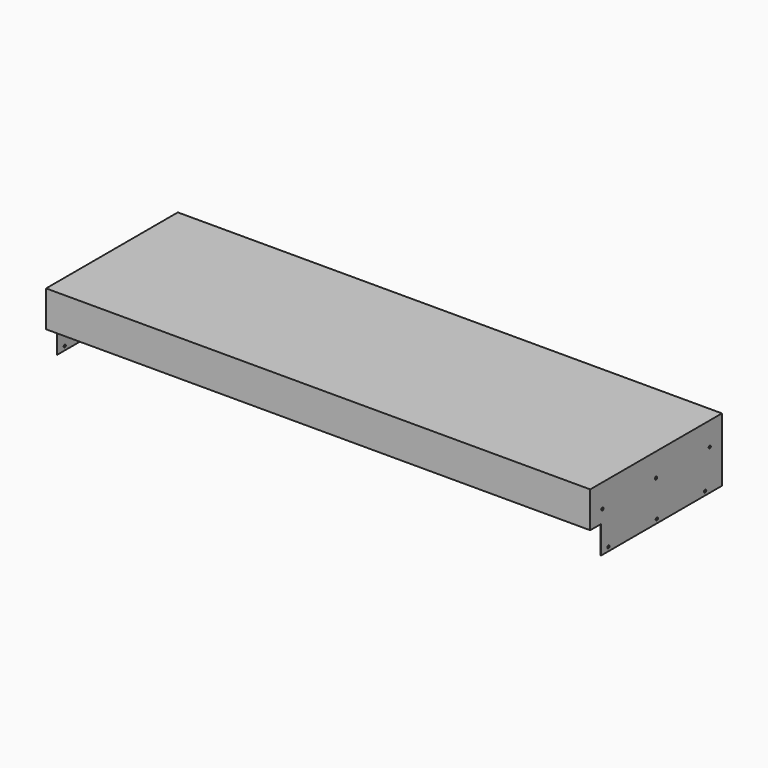
from build123d import *

# Parameters (mm, degrees)
F0_W     = 1029.208
F0_H     = 311.4294
F1_DEPTH = 120.65
F2_T     = -0.762
F3_W     = 25.4
F3_H     = 52.578
F4_DEPTH = 1029.209
F6_D     = 5.2197
F6_DEPTH = 1.016
F6_TIP   = 1.5681560866
F8_D     = 5.2197
F10_D    = 5.2197


# Not quite as in the source:
# - a feature names something its author has since deleted; it is built from what else it names


with BuildPart() as f1:
    # F0 (on Top) → F1 (new body)
    with BuildSketch(Plane.XY):
        Rectangle(F0_W, F0_H)
    extrude(amount=F1_DEPTH)

    # F2
    f2_openings = [f1.faces().sort_by_distance(p)[0] for p in [
        (0, 0, 0),
    ]]
    offset(amount=F2_T, openings=f2_openings)

    # F3 (on face) → F4 (cut, through all)
    with BuildSketch(Plane(origin=(-514.604, 0, 0), x_dir=(0, -1, 0), z_dir=(-1, 0, 0))):
        with Locations((143.0147, 26.289)):
            Rectangle(F3_W, F3_H)
    extrude(amount=-F4_DEPTH, mode=Mode.SUBTRACT)

    # F6
    with Locations(Plane(origin=(0, 155.7147, 0), x_dir=(-1, 0, 0), z_dir=(0, 1, 0))):
        with Locations((-488.95, 7.366), (488.95, 7.366), (0, 7.366), (-244.475, 7.366), (244.475, 7.366)):
            Hole(F6_D / 2, depth=F6_DEPTH)
            with Locations((0, 0, -(F6_DEPTH + F6_TIP / 2))):  # 118° drill point
                Cone(0, F6_D / 2, F6_TIP, mode=Mode.SUBTRACT)

    # F8 (through all)
    with Locations(Plane(origin=(-514.604, 0, 0), x_dir=(0, -1, 0), z_dir=(-1, 0, 0))):
        with Locations((-116.0907, 7.366), (-1.7907, 7.366), (112.5093, 7.366)):
            Hole(F8_D / 2)

    # F10 (through all)
    with Locations(Plane(origin=(-514.604, 0, 0), x_dir=(0, -1, 0), z_dir=(-1, 0, 0))):
        with Locations((-127, 76.2), (0, 76.2), (127, 76.2)):
            Hole(F10_D / 2)


solid = f1.part
